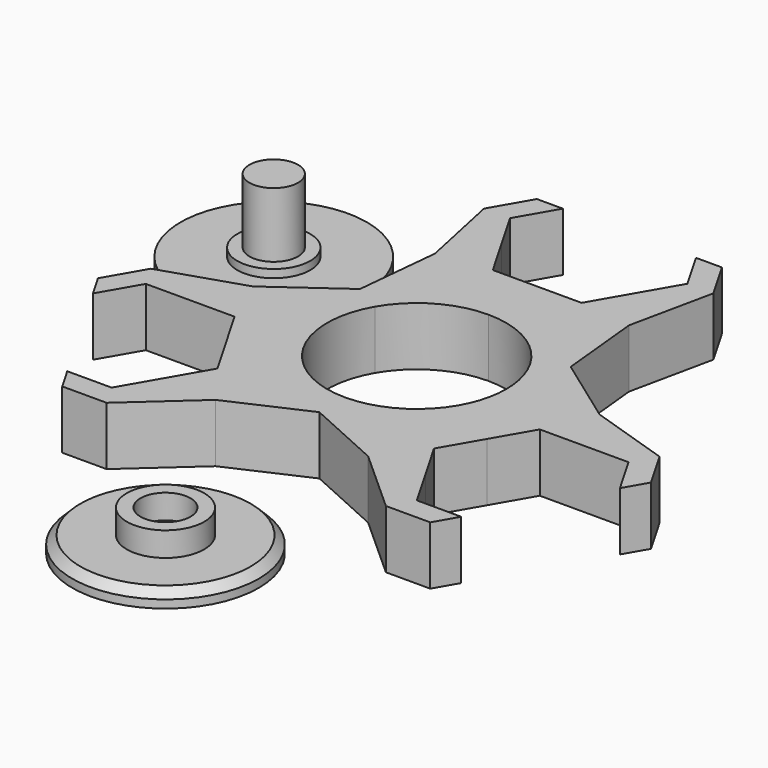
from build123d import *

# Parameters (mm, degrees)
F1_DEPTH  = 7.2
F2_R      = 11.5
F2_R_2    = 4.775
F3_DEPTH  = 2
F2_R_3    = 3.085
F4_DEPTH  = 5
F5_DEPTH  = 2
F2_R_4    = 4.5
F2_R_5    = 3
F6_DEPTH  = 3
F7_DEPTH  = 11
F8_DEPTH  = 2
F12_DEPTH = 25
F13_SIZE  = 1


# Not quite as in the source:
# - ends of sketch curves that miss each other by under 0.0002 mm in the source are joined


with BuildPart() as f1:
    # F0 (on Top) → F1 (new body)
    with BuildSketch(Plane.XY):
        with BuildLine():
            ThreePointArc((-9.5695807118, 5.525), (-5.525, 9.5695807118), (0, 11.05))
            Line((0, 11.05), (0, 15.8))
            Line((0, 15.8), (-7.0725407976, 15.8))
            Line((-7.0725407976, 15.8), (-10.6088111044, 21.9249998408))
            Line((-10.6088111044, 21.9249998408), (-11.4127894135, 23.3175311203))
            Line((-11.4127894135, 23.3175311203), (-11.965584329, 17.775))
            Line((-11.965584329, 17.775), (-12.9903810568, 7.5))
            Line((-12.9903810568, 7.5), (-9.5695807118, 5.525))
        make_face()
        with BuildLine():
            Line((-13.6832013798, -7.9), (-9.5695807118, -5.525))
            ThreePointArc((-9.5695807118, -5.525), (-11.05, 0), (-9.5695807118, 5.525))
            Line((-9.5695807118, 5.525), (-12.9903810568, 7.5))
            Line((-12.9903810568, 7.5), (-21.3763937167, 1.475))
            Line((-21.3763937167, 1.475), (-25.8999690105, -1.775))
            Line((-25.8999690105, -1.775), (-24.2920125762, -1.775))
            Line((-24.2920125762, -1.775), (-17.2194717786, -1.775))
            Line((-17.2194717786, -1.775), (-13.6832013798, -7.9))
        make_face()
        with BuildLine():
            ThreePointArc((-24.2920125762, -1.775), (-18.1670125219, -3.416188835), (-13.6832013171, -7.9000001085))
            Line((-13.6832013171, -7.9000001085), (-17.2194717786, -1.775))
            Line((-17.2194717786, -1.775), (-24.2920125762, -1.775))
        make_face()
        with BuildLine():
            Line((-16.0864218753, -9.2875), (-13.6832013798, -7.9))
            ThreePointArc((-13.6832013798, -7.9), (-18.1670125219, -3.416188835), (-24.2920125762, -1.775))
            ThreePointArc((-24.2920125762, -1.775), (-25.1900373543, -1.8079606083), (-26.0832295704, -1.9066650616))
            Line((-26.0832295704, -1.9066650616), (-29.7624063767, -4.55))
            Line((-29.7624063767, -4.55), (-24.2920125762, -4.55))
            Line((-24.2920125762, -4.55), (-18.8216187756, -4.55))
            Line((-18.8216187756, -4.55), (-16.0864218753, -9.2875))
        make_face()
        with BuildLine():
            ThreePointArc((-34.9008237666, -7.8999999897), (-31.1782445382, -3.8937459135), (-26.0832295704, -1.9066650616))
            Line((-26.0832295704, -1.9066650616), (-25.8999690105, -1.775))
            Line((-25.8999690105, -1.775), (-31.3645533737, -1.775))
            Line((-31.3645533737, -1.775), (-34.9008237666, -7.8999999897))
        make_face()
        with BuildLine():
            ThreePointArc((-34.900823478, -20.1500005101), (-36.5420125762, -14.0250002885), (-34.9008237666, -7.8999999897))
            Line((-34.9008237666, -7.8999999897), (-38.4370941713, -14.025))
            Line((-38.4370941713, -14.025), (-34.900823478, -20.1500005101))
        make_face()
        with BuildLine():
            Line((-29.7624063767, -4.55), (-26.0832295704, -1.9066650616))
            ThreePointArc((-26.0832295704, -1.9066650616), (-31.1782445382, -3.8937459135), (-34.9008237666, -7.8999999897))
            ThreePointArc((-34.9008237666, -7.8999999897), (-36.5420125762, -14.0250002885), (-34.900823478, -20.1500005101))
            ThreePointArc((-34.900823478, -20.1500005101), (-30.4170123211, -24.6338113436), (-24.2920125762, -26.275))
            ThreePointArc((-24.2920125762, -26.275), (-18.9612051515, -25.0542788613), (-14.692835165, -21.6354068899))
            Line((-14.692835165, -21.6354068899), (-18.8216187756, -23.5))
            Line((-18.8216187756, -23.5), (-24.2920125762, -23.5))
            Line((-24.2920125762, -23.5), (-29.7624063767, -23.5))
            Line((-29.7624063767, -23.5), (-32.4976032385, -18.7625000667))
            Line((-32.4976032385, -18.7625000667), (-35.2328001773, -14.025))
            Line((-35.2328001773, -14.025), (-32.4976032385, -9.2874999333))
            Line((-32.4976032385, -9.2874999333), (-29.7624063767, -4.55))
        make_face()
        with BuildLine():
            Line((-31.3645533737, -26.275), (-24.2920125762, -26.275))
            ThreePointArc((-24.2920125762, -26.275), (-30.4170123211, -24.6338113436), (-34.900823478, -20.1500005101))
            Line((-34.900823478, -20.1500005101), (-31.3645533737, -26.275))
        make_face()
        with BuildLine():
            Line((-17.2194717786, -26.275), (-14.487179597, -21.5425311203))
            Line((-14.487179597, -21.5425311203), (-14.692835165, -21.6354068899))
            ThreePointArc((-14.692835165, -21.6354068899), (-18.9612051515, -25.0542788613), (-24.2920125762, -26.275))
            Line((-24.2920125762, -26.275), (-17.2194717786, -26.275))
        make_face()
        with BuildLine():
            ThreePointArc((-12.0420125762, -14.025), (-12.4594211879, -10.854466758), (-13.6832013171, -7.9000001085))
            Line((-13.6832013171, -7.9000001085), (-16.0864218753, -9.2875))
            Line((-16.0864218753, -9.2875), (-13.351224975, -14.025))
            Line((-13.351224975, -14.025), (-16.0864219138, -18.7625000667))
            Line((-16.0864219138, -18.7625000667), (-18.8216187756, -23.5))
            Line((-18.8216187756, -23.5), (-14.692835165, -21.6354068899))
            ThreePointArc((-14.692835165, -21.6354068899), (-14.1607584743, -20.9112319395), (-13.6832013466, -20.1499999424))
            ThreePointArc((-13.6832013466, -20.1499999424), (-12.4594211955, -17.1955332704), (-12.0420125762, -14.025))
        make_face()
        Polygon((-17.2194717786, -26.275), (-9.4108093878, -19.25), (-14.487179597, -21.5425311203), align=None)
        with BuildLine():
            Line((0, -15), (0, -11.05))
            ThreePointArc((0, -11.05), (-5.525, -9.5695807118), (-9.5695807118, -5.525))
            Line((-9.5695807118, -5.525), (-13.6832013798, -7.9))
            Line((-13.6832013798, -7.9), (-10.146930981, -14.025))
            Line((-10.146930981, -14.025), (-13.6832013466, -20.1499999424))
            Line((-13.6832013466, -20.1499999424), (-14.487179597, -21.5425311203))
            Line((-14.487179597, -21.5425311203), (-9.4108093878, -19.25))
            Line((-9.4108093878, -19.25), (0, -15))
        make_face()
        with BuildLine():
            Line((-14.692835165, -21.6354068899), (-14.487179597, -21.5425311203))
            Line((-14.487179597, -21.5425311203), (-13.6832013466, -20.1499999424))
            ThreePointArc((-13.6832013466, -20.1499999424), (-14.1607584743, -20.9112319395), (-14.692835165, -21.6354068899))
        make_face()
        with BuildLine():
            ThreePointArc((-26.0832295704, -1.9066650616), (-25.1900373543, -1.8079606083), (-24.2920125762, -1.775))
            Line((-24.2920125762, -1.775), (-25.8999690105, -1.775))
            Line((-25.8999690105, -1.775), (-26.0832295704, -1.9066650616))
        make_face()
        with BuildLine():
            Line((-10.146930981, -14.025), (-13.6832013171, -7.9000001085))
            ThreePointArc((-13.6832013171, -7.9000001085), (-12.4594211879, -10.854466758), (-12.0420125762, -14.025))
            ThreePointArc((-12.0420125762, -14.025), (-12.4594211955, -17.1955332704), (-13.6832013466, -20.1499999424))
            Line((-13.6832013466, -20.1499999424), (-10.146930981, -14.025))
        make_face()
        with BuildLine():
            Line((13.6832013798, -7.9), (9.5695807118, -5.525))
            ThreePointArc((9.5695807118, -5.525), (5.525, -9.5695807118), (0, -11.05))
            Line((0, -11.05), (0, -15))
            Line((0, -15), (9.4108093878, -19.25))
            Line((9.4108093878, -19.25), (14.487179597, -21.5425311203))
            Line((14.487179597, -21.5425311203), (13.6832016265, -20.1500004272))
            Line((13.6832016265, -20.1500004272), (10.146930981, -14.025))
            Line((10.146930981, -14.025), (13.6832013838, -7.8999999931))
        make_face()
        with BuildLine():
            ThreePointArc((11.05, 0), (10.6734803805, -2.8599504484), (9.5695807118, -5.525))
            Line((9.5695807118, -5.525), (13.6832013798, -7.9))
            Line((13.6832013838, -7.8999999931), (17.2194717786, -1.775))
            Line((17.2194717786, -1.775), (24.2920125762, -1.775))
            Line((24.2920125762, -1.775), (25.8999690105, -1.775))
            Line((25.8999690105, -1.775), (21.3763937167, 1.475))
            Line((21.3763937167, 1.475), (12.9903810568, 7.5))
            Line((12.9903810568, 7.5), (9.5695807118, 5.525))
            ThreePointArc((9.5695807118, 5.525), (10.6734803805, 2.8599504484), (11.05, 0))
        make_face()
        with BuildLine():
            ThreePointArc((0, 11.05), (5.525, 9.5695807118), (9.5695807118, 5.525))
            Line((9.5695807118, 5.525), (12.9903810568, 7.5))
            Line((12.9903810568, 7.5), (11.965584329, 17.775))
            Line((11.965584329, 17.775), (11.4127894135, 23.3175311203))
            Line((11.4127894135, 23.3175311203), (10.6088112296, 21.9250000576))
            Line((10.6088112296, 21.9250000576), (7.0725407976, 15.8))
            Line((7.0725407976, 15.8), (0, 15.8))
            Line((0, 15.8), (0, 11.05))
        make_face()
        with BuildLine():
            ThreePointArc((13.6832016265, -20.1500004272), (12.0420125762, -14.0250002427), (13.6832013838, -7.8999999931))
            Line((13.6832013838, -7.8999999931), (10.146930981, -14.025))
            Line((10.146930981, -14.025), (13.6832016265, -20.1500004272))
        make_face()
        with BuildLine():
            Line((16.0864218753, -9.2875), (13.6832013798, -7.9))
            ThreePointArc((13.6832013838, -7.8999999931), (12.0420125762, -14.0250002427), (13.6832016265, -20.1500004272))
            ThreePointArc((13.6832016265, -20.1500004272), (14.1607586317, -20.911232171), (14.692835165, -21.6354068899))
            Line((14.692835165, -21.6354068899), (18.8216187756, -23.5))
            Line((18.8216187756, -23.5), (16.0864219138, -18.7625000667))
            Line((16.0864219138, -18.7625000667), (13.351224975, -14.025))
            Line((13.351224975, -14.025), (16.0864218881, -9.2874999778))
        make_face()
        with BuildLine():
            ThreePointArc((24.2920125762, -1.775), (18.1670125796, -3.4161888017), (13.6832013838, -7.8999999931))
            Line((13.6832013798, -7.9), (16.0864218753, -9.2875))
            Line((16.0864218881, -9.2874999778), (18.8216187756, -4.55))
            Line((18.8216187756, -4.55), (24.2920125762, -4.55))
            Line((24.2920125762, -4.55), (29.7624063767, -4.55))
            Line((29.7624063767, -4.55), (26.0832295704, -1.9066650616))
            ThreePointArc((26.0832295704, -1.9066650616), (25.1900373543, -1.8079606083), (24.2920125762, -1.775))
        make_face()
        with BuildLine():
            Line((17.2194717786, -1.775), (13.6832013838, -7.8999999931))
            ThreePointArc((13.6832013838, -7.8999999931), (18.1670125796, -3.4161888017), (24.2920125762, -1.775))
            Line((24.2920125762, -1.775), (17.2194717786, -1.775))
        make_face()
        with BuildLine():
            ThreePointArc((14.692835165, -21.6354068899), (14.1607586317, -20.911232171), (13.6832016265, -20.1500004272))
            Line((13.6832016265, -20.1500004272), (14.487179597, -21.5425311203))
            Line((14.487179597, -21.5425311203), (14.692835165, -21.6354068899))
        make_face()
        Polygon((14.487179597, -21.5425311203), (9.4108093878, -19.25), (17.2194717786, -26.275), align=None)
        with BuildLine():
            ThreePointArc((24.2920125762, -26.275), (18.9612051515, -25.0542788613), (14.692835165, -21.6354068899))
            Line((14.692835165, -21.6354068899), (14.487179597, -21.5425311203))
            Line((14.487179597, -21.5425311203), (17.2194717786, -26.275))
            Line((17.2194717786, -26.275), (24.2920125762, -26.275))
        make_face()
        with BuildLine():
            ThreePointArc((34.9008238058, -7.9000000576), (31.1782445706, -3.8937459356), (26.0832295704, -1.9066650616))
            Line((26.0832295704, -1.9066650616), (29.7624063767, -4.55))
            Line((29.7624063767, -4.55), (32.4976033488, -9.2875001244))
            Line((32.4976033488, -9.2875001244), (35.2328001773, -14.025))
            Line((35.2328001773, -14.025), (32.4976032385, -18.7625000667))
            Line((32.4976032385, -18.7625000667), (29.7624063767, -23.5))
            Line((29.7624063767, -23.5), (24.2920125762, -23.5))
            Line((24.2920125762, -23.5), (18.8216187756, -23.5))
            Line((18.8216187756, -23.5), (14.692835165, -21.6354068899))
            ThreePointArc((14.692835165, -21.6354068899), (18.9612051515, -25.0542788613), (24.2920125762, -26.275))
            ThreePointArc((24.2920125762, -26.275), (30.4170126049, -24.6338111797), (34.9008238058, -20.1499999424))
            ThreePointArc((34.9008238058, -20.1499999424), (36.1246039568, -17.1955332704), (36.5420125762, -14.025))
            ThreePointArc((36.5420125762, -14.025), (36.1246039568, -10.8544667296), (34.9008238058, -7.9000000576))
        make_face()
        with BuildLine():
            ThreePointArc((34.9008238058, -20.1499999424), (30.4170126049, -24.6338111797), (24.2920125762, -26.275))
            Line((24.2920125762, -26.275), (31.3645533737, -26.275))
            Line((31.3645533737, -26.275), (34.9008238058, -20.1499999424))
        make_face()
        with BuildLine():
            Line((38.4370941713, -14.025), (34.9008238058, -7.9000000576))
            ThreePointArc((34.9008238058, -7.9000000576), (36.1246039568, -10.8544667296), (36.5420125762, -14.025))
            ThreePointArc((36.5420125762, -14.025), (36.1246039568, -17.1955332704), (34.9008238058, -20.1499999424))
            Line((34.9008238058, -20.1499999424), (38.4370941713, -14.025))
        make_face()
        with BuildLine():
            Line((25.8999690105, -1.775), (26.0832295704, -1.9066650616))
            ThreePointArc((26.0832295704, -1.9066650616), (31.1782445706, -3.8937459356), (34.9008238058, -7.9000000576))
            Line((34.9008238058, -7.9000000576), (31.3645533737, -1.775))
            Line((31.3645533737, -1.775), (25.8999690105, -1.775))
        make_face()
        with BuildLine():
            Line((25.8999690105, -1.775), (24.2920125762, -1.775))
            ThreePointArc((24.2920125762, -1.775), (25.1900373543, -1.8079606083), (26.0832295704, -1.9066650616))
            Line((26.0832295704, -1.9066650616), (25.8999690105, -1.775))
        make_face()
        Polygon((-25.8999690105, -1.775), (-21.3763937167, 1.475), (-31.3645533737, -1.775), align=None)
        Polygon((21.3763937167, 1.475), (25.8999690105, -1.775), (31.3645533737, -1.775), align=None)
        Polygon((11.4127894135, 23.3175311203), (11.965584329, 17.775), (14.1450815951, 28.05), align=None)
        Polygon((-14.1450815951, 28.05), (-11.965584329, 17.775), (-11.4127894135, 23.3175311203), align=None)
        with BuildLine():
            ThreePointArc((-10.6088111044, 21.9249998408), (-6.1249999204, 17.4411887577), (0, 15.8))
            Line((0, 15.8), (0, 18.575))
            Line((0, 18.575), (-5.4703938006, 18.575))
            Line((-5.4703938006, 18.575), (-8.2055907888, 23.3125001523))
            Line((-8.2055907888, 23.3125001523), (-10.9407876011, 28.05))
            Line((-10.9407876011, 28.05), (-11.3903944054, 23.5420719515))
            ThreePointArc((-11.3903944054, 23.5420719515), (-11.0292788213, 22.7191924925), (-10.6088111044, 21.9249998408))
        make_face()
        with BuildLine():
            Line((-7.0725407976, 15.8), (0, 15.8))
            ThreePointArc((0, 15.8), (-6.1249999204, 17.4411887577), (-10.6088111044, 21.9249998408))
            Line((-10.6088111044, 21.9249998408), (-7.0725407976, 15.8))
        make_face()
        with BuildLine():
            Line((0, 18.575), (0, 15.8))
            ThreePointArc((0, 15.8), (6.1250000288, 17.4411888203), (10.6088112296, 21.9250000576))
            ThreePointArc((10.6088112296, 21.9250000576), (11.0292788758, 22.7191926052), (11.3903944054, 23.5420719515))
            Line((11.3903944054, 23.5420719515), (10.9407876011, 28.05))
            Line((10.9407876011, 28.05), (8.2055905941, 23.3124998151))
            Line((8.2055905941, 23.3124998151), (5.4703938006, 18.575))
            Line((5.4703938006, 18.575), (0, 18.575))
        make_face()
        with BuildLine():
            ThreePointArc((10.6088112296, 21.9250000576), (6.1250000288, 17.4411888203), (0, 15.8))
            Line((0, 15.8), (7.0725407976, 15.8))
            Line((7.0725407976, 15.8), (10.6088112296, 21.9250000576))
        make_face()
        with BuildLine():
            Line((11.3903944054, 23.5420719515), (11.4127894135, 23.3175311203))
            Line((11.4127894135, 23.3175311203), (14.1450815951, 28.05))
            Line((14.1450815951, 28.05), (10.6088112296, 34.1749999424))
            ThreePointArc((10.6088112296, 34.1749999424), (11.8325913806, 31.2205332704), (12.25, 28.05))
            ThreePointArc((12.25, 28.05), (12.0331797848, 25.7554228566), (11.3903944054, 23.5420719515))
        make_face()
        with BuildLine():
            ThreePointArc((-10.6088111044, 34.1750001592), (-12.2170393849, 28.9480248699), (-11.3903944054, 23.5420719515))
            Line((-11.3903944054, 23.5420719515), (-10.9407876011, 28.05))
            Line((-10.9407876011, 28.05), (-8.2055906623, 32.7875000667))
            Line((-8.2055906623, 32.7875000667), (-5.4703938006, 37.525))
            Line((-5.4703938006, 37.525), (0, 37.525))
            Line((0, 37.525), (5.4703938006, 37.525))
            Line((5.4703938006, 37.525), (8.2055906746, 32.7875000454))
            Line((8.2055906746, 32.7875000454), (10.9407876011, 28.05))
            Line((10.9407876011, 28.05), (11.3903944054, 23.5420719515))
            ThreePointArc((11.3903944054, 23.5420719515), (12.0331797848, 25.7554228566), (12.25, 28.05))
            ThreePointArc((12.25, 28.05), (11.8325913806, 31.2205332704), (10.6088112296, 34.1749999424))
            ThreePointArc((10.6088112296, 34.1749999424), (6.1250000288, 38.6588111797), (0, 40.3))
            ThreePointArc((0, 40.3), (-6.1249999204, 38.6588112423), (-10.6088111044, 34.1750001592))
        make_face()
        with BuildLine():
            ThreePointArc((0, 40.3), (6.1250000288, 38.6588111797), (10.6088112296, 34.1749999424))
            Line((10.6088112296, 34.1749999424), (7.0725407976, 40.3))
            Line((7.0725407976, 40.3), (0, 40.3))
        make_face()
        with BuildLine():
            Line((-7.0725407976, 40.3), (-10.6088111044, 34.1750001592))
            ThreePointArc((-10.6088111044, 34.1750001592), (-6.1249999204, 38.6588112423), (0, 40.3))
            Line((0, 40.3), (-7.0725407976, 40.3))
        make_face()
        with BuildLine():
            Line((-11.4127894135, 23.3175311203), (-11.3903944054, 23.5420719515))
            ThreePointArc((-11.3903944054, 23.5420719515), (-12.2170393849, 28.9480248699), (-10.6088111044, 34.1750001592))
            Line((-10.6088111044, 34.1750001592), (-14.1450815951, 28.05))
            Line((-14.1450815951, 28.05), (-11.4127894135, 23.3175311203))
        make_face()
        with BuildLine():
            Line((-11.4127894135, 23.3175311203), (-10.6088111044, 21.9249998408))
            ThreePointArc((-10.6088111044, 21.9249998408), (-11.0292788213, 22.7191924925), (-11.3903944054, 23.5420719515))
            Line((-11.3903944054, 23.5420719515), (-11.4127894135, 23.3175311203))
        make_face()
        with BuildLine():
            ThreePointArc((11.3903944054, 23.5420719515), (11.0292788758, 22.7191926052), (10.6088112296, 21.9250000576))
            Line((10.6088112296, 21.9250000576), (11.4127894135, 23.3175311203))
            Line((11.4127894135, 23.3175311203), (11.3903944054, 23.5420719515))
        make_face()
    extrude(amount=F1_DEPTH)

    # F11 (on face) → F12 (cut)
    with BuildSketch(Plane.XY.offset(7.2)):
        Polygon((-32.497603277, -9.2875), (-34.099750274, -6.5125), (-38.4370941713, -14.025), (-31.3645533737, -26.275), (-22.6898655792, -26.275), (-24.2920125762, -23.5), (-29.7624063767, -23.5), (-35.2328001773, -14.025), align=None)
        Polygon((-11.4098846949, 32.7875), (-8.2055907009, 32.7875), (-5.4703938006, 37.525), (5.4703938006, 37.525), (8.2055907009, 32.7875), (11.4098846949, 32.7875), (7.0725407976, 40.3), (-7.0725407976, 40.3), align=None)
        Polygon((38.4370941713, -14.025), (34.099750274, -6.5125), (32.497603277, -9.2875), (35.2328001773, -14.025), (29.7624063767, -23.5), (24.2920125762, -23.5), (22.6898655792, -26.275), (31.3645533737, -26.275), align=None)
    extrude(amount=-F12_DEPTH, mode=Mode.SUBTRACT)


with BuildPart() as f3:
    # F2 (on Top) → F3 (new body)
    with BuildSketch(Plane.XY):
        with Locations((-37.296205759, -49.7740730643)):
            Circle(F2_R)
        with Locations((-37.296205759, -49.7740730643)):
            Circle(F2_R_2, mode=Mode.SUBTRACT)
    extrude(amount=F3_DEPTH)

    # F2 (on Top) → F4 (join)
    with BuildSketch(Plane.XY):
        with Locations((-37.296205759, -49.7740730643)):
            Circle(F2_R_2)
        with Locations((-37.296205759, -49.7740730643)):
            Circle(F2_R_3, mode=Mode.SUBTRACT)
    extrude(amount=F4_DEPTH)

    # F2 (on Top) → F5 (join)
    with BuildSketch(Plane.XY):
        with Locations((-37.296205759, -49.7740730643)):
            Circle(F2_R_3)
    extrude(amount=F5_DEPTH)


with BuildPart() as f6:
    # F2 (on Top) → F6 (new body)
    with BuildSketch(Plane.XY):
        with Locations((-46.9284579158, 47.9787290096)):
            Circle(F2_R_4)
        with Locations((-46.9284579158, 47.9787290096)):
            Circle(F2_R_5, mode=Mode.SUBTRACT)
    extrude(amount=F6_DEPTH)

    # F2 (on Top) → F7 (join)
    with BuildSketch(Plane.XY):
        with Locations((-46.9284579158, 47.9787290096)):
            Circle(F2_R_5)
    extrude(amount=F7_DEPTH)

    # F2 (on Top) → F8 (join)
    with BuildSketch(Plane.XY):
        with Locations((-46.9284579158, 47.9787290096)):
            Circle(F2_R)
        with Locations((-46.9284579158, 47.9787290096)):
            Circle(F2_R_4, mode=Mode.SUBTRACT)
    extrude(amount=F8_DEPTH)


with BuildPart() as f3_1:
    # F9: moved
    add(f3.part.moved(Location((35.5, 13.3, 0))))

    # F13
    f13_edges = [f3_1.edges().sort_by_distance(p)[0] for p in [
        (-13.296206, -36.474073, 2),
    ]]
    chamfer(f13_edges, length=F13_SIZE)


with BuildPart() as f6_1:
    # F10: moved
    add(f6.part.moved(Location((17, -32.6, 0))))


solid = Compound([f1.part, f3_1.part, f6_1.part])
